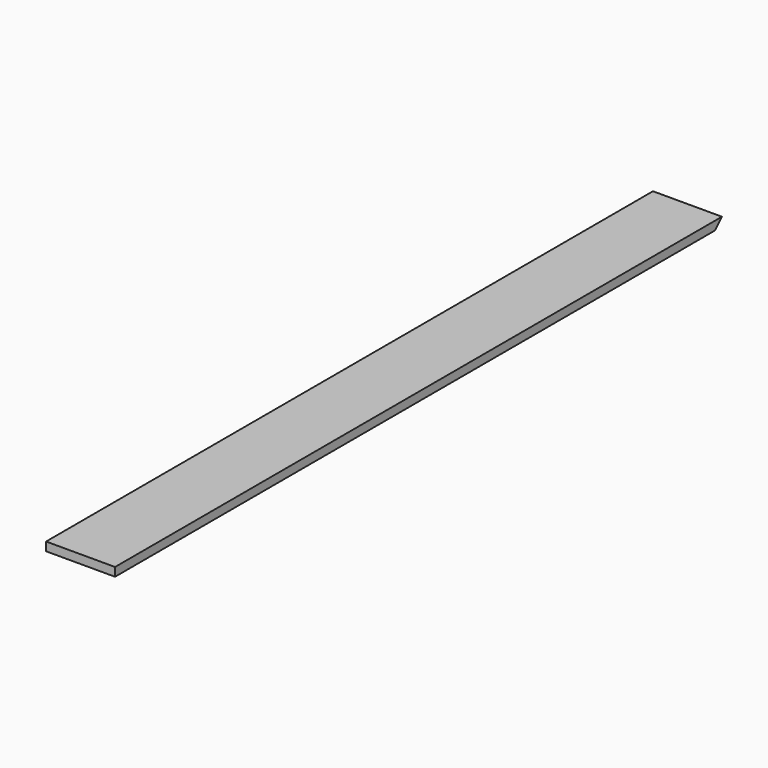
from build123d import *

# Parameters (mm, degrees)
F0_W     = 279.4
F0_H     = 3.175
F1_DEPTH = 25.4
F2_SIZE  = 3.17499


# Not quite as in the source:
# - a fillet or chamfer is up to 0.001 mm smaller than in the source, because OpenCascade refuses the exact size


with BuildPart() as f1:
    # F0 (on Right) → F1 (new body)
    with BuildSketch(Plane.YZ):
        with Locations((-139.7, 1.5875)):
            Rectangle(F0_W, F0_H)
    extrude(amount=F1_DEPTH)

    # F2 (size 3.175 in the source; OpenCascade refuses exactly that, so slightly less here)
    f2_edges = [f1.edges().sort_by_distance(p)[0] for p in [
        (12.7, 0, 0),
    ]]
    chamfer(f2_edges, length=F2_SIZE)


solid = f1.part
